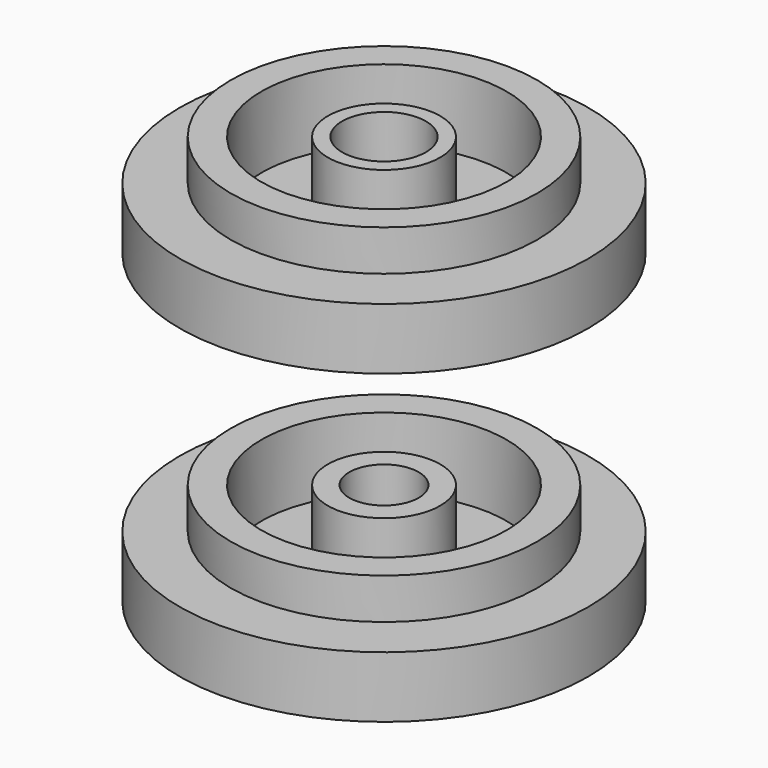
from build123d import *

# Parameters (mm, degrees)
F0_W     = 7.5
F0_H     = 2
F2_T     = 1.5
F3_R     = 2.75
F4_DEPTH = 3.5
F5_R     = 1.7
F8_DEPTH = 5
F7_R     = 2.05
F9_DEPTH = 5


# Not quite as in the source:
# - a shell that OpenCascade refuses in one call is made with other operations: the cavity is built on its own and cut out


with BuildPart() as f1:
    # F0 (on Right) → F1 (revolve)
    with BuildSketch(Plane.YZ):
        with Locations((-3.75, 1)):
            Rectangle(F0_W, F0_H)
        Polygon((0, 0), (-7.5, 0), (-10, 0), (-10, -3), (0, -3), align=None)
    revolve(axis=Axis((0, 0, 1), (0, 0, -1)))

    # F2: shell of thickness 1.5, made by hand


with BuildPart() as f2_core1:
    # F2_t2: copy of F1
    add(f1.part)

    # the walls: a layer under each face that stays
    f2_faces = [f2_core1.faces().sort_by_distance(p)[0] for p in [
        (0, 7.5, 1),
        (6.6666666667, -6.6666666667, 0),
        (0, 10, -1.5),
        (0, 0, -3),
    ]]
    thicken(f2_faces, amount=-F2_T, mode=Mode.SUBTRACT)

    # F2_s3 → F2_t4 (revolve, cut)
    with BuildSketch(Plane.YZ):
        Polygon((-7.515, 0.015), (-6, 0), (-6, -1.5), (-7.5, -1.5), align=None)
    revolve(axis=Axis((0, 0, 0), (0, 0, -1)), mode=Mode.SUBTRACT)


with BuildPart() as f1_1:
    add(f1.part)

    # what is left inside the walls is the cavity
    f2_cavity = [f2_core1.part.solids().sort_by_distance(p)[0] for p in [
        (0, 5.985, 0.833333),
    ]]
    add(f2_cavity, mode=Mode.SUBTRACT)

    # F3 (on face) → F4 (join, through all)
    with BuildSketch(Plane.XY.offset(-1.5)):
        Circle(F3_R)
    extrude(amount=F4_DEPTH)


with BuildPart() as f6_1:
    # F6: copy of F1
    add(f1_1.part.moved(Location((0, 0, 15))))

    # F7 (on face) → F9 (cut, through all)
    with BuildSketch(Plane.XY.offset(17)):
        Circle(F7_R)
    extrude(amount=-F9_DEPTH, mode=Mode.SUBTRACT)


with BuildPart() as f1_2:
    add(f1_1.part)

    # F5 (on face) → F8 (cut, through all)
    with BuildSketch(Plane.XY.offset(2)):
        Circle(F5_R)
    extrude(amount=-F8_DEPTH, mode=Mode.SUBTRACT)


solid = Compound([f6_1.part, f1_2.part])
